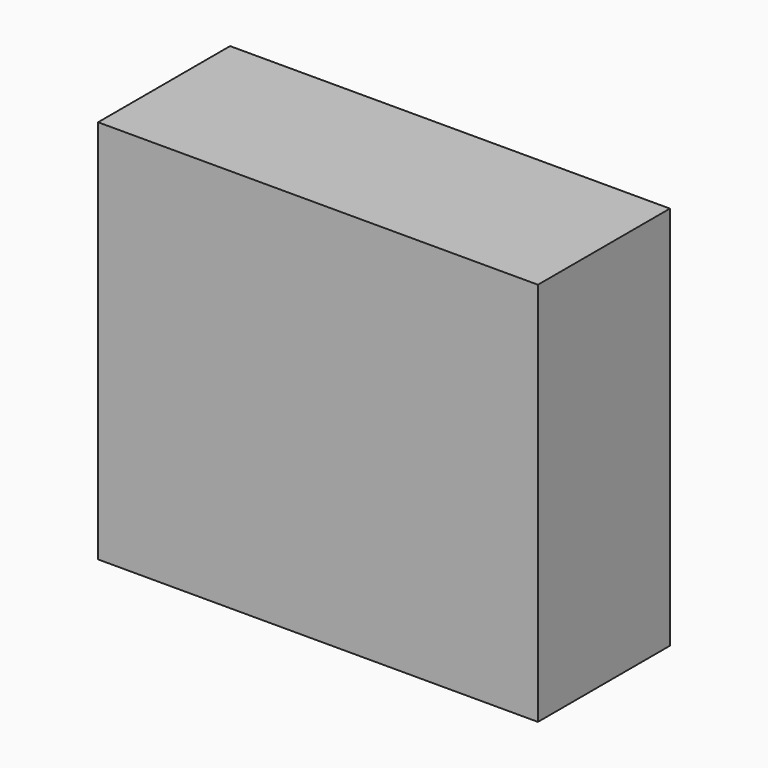
from build123d import *

# Parameters (mm, degrees)
F0_W        = 50.8
F0_H        = 19.05
F1_DEPTH    = 44.45
F2_W        = 3.81
F2_H        = 6.35
F3_DEPTH    = 5.08
F4_R        = 1.0795
F5_DEPTH    = 1.27
F6_R        = 1.0795
F7_DEPTH    = 1.27
F8_T        = 1.27
F8_T3_DEPTH = 6.35
F8_T5_DEPTH = 7.62
F8_T7_DEPTH = 8.89
F9_DEPTH    = 2.54


# Not quite as in the source:
# - a shell that OpenCascade refuses in one call is made with other operations: the cavity is built on its own and cut out


with BuildPart() as f1:
    # F0 (on Top) → F1 (new body)
    with BuildSketch(Plane.XY):
        Rectangle(F0_W, F0_H)
    extrude(amount=F1_DEPTH)

    # F2 (on face) → F3 (cut)
    with BuildSketch(Plane(origin=(0, 0, 0), x_dir=(1, 0, 0), z_dir=(0, 0, -1))):
        with Locations((-23.495, 0)):
            Rectangle(F2_W, F2_H)
    extrude(amount=-F3_DEPTH, mode=Mode.SUBTRACT)

    # F4 (on face) → F5 (cut)
    with BuildSketch(Plane.XZ.offset(-3.175)):
        with Locations((-23.495, 2.54)):
            Circle(F4_R)
    extrude(amount=-F5_DEPTH, mode=Mode.SUBTRACT)

    # F6 (on face) → F7 (cut)
    with BuildSketch(Plane(origin=(0, -3.175, 0), x_dir=(-1, 0, 0), z_dir=(0, 1, 0))):
        with Locations((23.495, 2.54)):
            Circle(F6_R)
    extrude(amount=-F7_DEPTH, mode=Mode.SUBTRACT)

    # F8: shell of thickness 1.27, made by hand


with BuildPart() as f8_core1:
    # F8_t2: copy of F1
    add(f1.part)

    # the walls: a layer under each face that stays
    f8_faces = [f8_core1.faces().sort_by_distance(p)[0] for p in [
        (0, -9.525, 22.225),
        (-25.4, 0, 22.225),
        (25.4, 0, 22.225),
        (0, 0, 44.45),
        (-24.765, 3.175, 4.2333333333),
        (-23.495, 0, 5.08),
        (-22.225, -3.175, 4.2333333333),
        (0, 9.525, 22.225),
        (-21.59, 0, 2.54),
        (-24.5745, 3.81, 2.54),
        (-22.4155, -3.81, 2.54),
        (-23.495, 4.445, 2.54),
        (-23.495, -4.445, 2.54),
    ]]
    thicken(f8_faces, amount=-F8_T, mode=Mode.SUBTRACT)

    # F8_s4 → F8_t3 (cut)
    with BuildSketch(Plane.YZ.offset(-26.67)):
        Polygon((3.1623, 5.0673), (4.445, 5.08), (4.445, 6.35), (3.175, 6.35), align=None)
        Polygon((-3.1623, 5.0673), (-3.175, 6.35), (-4.445, 6.35), (-4.445, 5.08), align=None)
    extrude(amount=F8_T3_DEPTH, mode=Mode.SUBTRACT)

    # F8_s6 → F8_t5 (cut)
    with BuildSketch(Plane.XY.offset(-1.27)):
        Polygon((-21.6027, 3.1623), (-21.59, 4.445), (-20.32, 4.445), (-20.32, 3.175), align=None)
        Polygon((-21.6027, -3.1623), (-21.59, -4.445), (-20.32, -4.445), (-20.32, -3.175), align=None)
    extrude(amount=F8_T5_DEPTH, mode=Mode.SUBTRACT)

    # F8_s8 → F8_t7 (cut)
    with BuildSketch(Plane.XZ.offset(-4.445)):
        Polygon((-21.6027, 5.0673), (-21.59, 6.35), (-20.32, 6.35), (-20.32, 5.08), align=None)
    extrude(amount=F8_T7_DEPTH, mode=Mode.SUBTRACT)

    # F8_s9 → F8_t10 (revolve, cut)
    with BuildSketch(Plane.XY.offset(2.54)):
        Polygon((-22.4282, 4.4323), (-21.1455, 4.445), (-21.1455, 5.715), (-22.4155, 5.715), align=None)
    revolve(axis=Axis((-23.495, 4.445, 2.54), (0, -1, 0)), mode=Mode.SUBTRACT)

    # F8_s11 → F8_t12 (revolve, cut)
    with BuildSketch(Plane.XY.offset(2.54)):
        Polygon((-24.5618, -4.4323), (-25.8445, -4.445), (-25.8445, -5.715), (-24.5745, -5.715), align=None)
    revolve(axis=Axis((-23.495, -4.445, 2.54), (0, 1, 0)), mode=Mode.SUBTRACT)


with BuildPart() as f1_1:
    add(f1.part)

    # what is left inside the walls is the cavity
    f8_cavity = [f8_core1.part.solids().sort_by_distance(p)[0] for p in [
        (0, -8.2423, 28.786667),
    ]]
    add(f8_cavity, mode=Mode.SUBTRACT)

    # F9 (add): a face of the model
    f9_faces = [f1_1.faces().sort_by_distance(p)[0] for p in [
        (-24.13, 0, 23.5412296588),
    ]]
    extrude(f9_faces, amount=F9_DEPTH)


solid = f1_1.part
